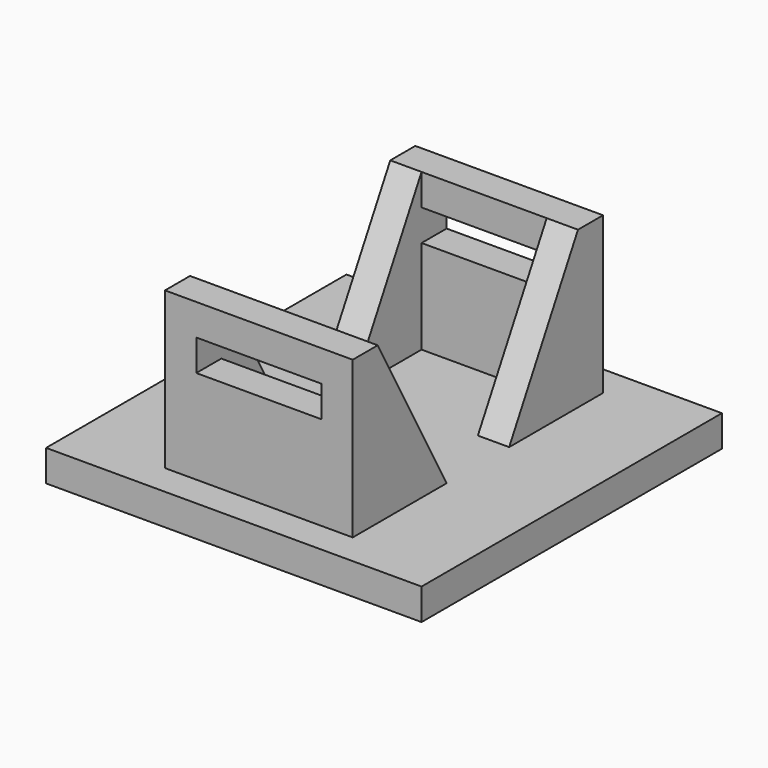
from build123d import *

# Parameters (mm, degrees)
F0_W     = 24
F0_H     = 24
F1_DEPTH = 2
F2_DEPTH = 10
F3_SIZE2 = 9.99999
F3_SIZE  = 5.49999
F4_SIZE2 = 9.99999
F4_SIZE  = 5.49999
F5_W     = 8
F5_H     = 2
F6_DEPTH = 25


# Not quite as in the source:
# - a fillet or chamfer is up to 0.001 mm smaller than in the source, because OpenCascade refuses the exact size


with BuildPart() as f1:
    # F0 (on Top) → F1 (new body)
    with BuildSketch(Plane.XY):
        Rectangle(F0_W, F0_H)
        Polygon((-6, -10), (-6, -2.5), (-4, -2.5), (-4, -8), (0, -8), (4, -8), (4, -2.5), (6, -2.5), (6, -10), (0, -10), align=None, mode=Mode.SUBTRACT)
        Polygon((-4, 2.5), (-6, 2.5), (-6, 10), (0, 10), (6, 10), (6, 2.5), (4, 2.5), (4, 8), (0, 8), (-4, 8), align=None, mode=Mode.SUBTRACT)
        Polygon((-6, 10), (-6, 2.5), (-4, 2.5), (-4, 8), (0, 8), (4, 8), (4, 2.5), (6, 2.5), (6, 10), (0, 10), align=None)
        Polygon((-4, -2.5), (-6, -2.5), (-6, -10), (0, -10), (6, -10), (6, -2.5), (4, -2.5), (4, -8), (0, -8), (-4, -8), align=None)
    extrude(amount=-F1_DEPTH)

    # F0 (on Top) → F2 (join)
    with BuildSketch(Plane.XY):
        Polygon((-6, 10), (-6, 2.5), (-4, 2.5), (-4, 8), (0, 8), (4, 8), (4, 2.5), (6, 2.5), (6, 10), (0, 10), align=None)
        Polygon((-4, -2.5), (-6, -2.5), (-6, -10), (0, -10), (6, -10), (6, -2.5), (4, -2.5), (4, -8), (0, -8), (-4, -8), align=None)
    extrude(amount=F2_DEPTH)

    # F3 (size 5.5 and 10 in the source; OpenCascade refuses exactly that, so slightly less here)
    f3_edges = [f1.edges().sort_by_distance(p)[0] for p in [
        (-5, 2.5, 10),
        (5, 2.5, 10),
    ]]
    f3_side = f1.faces().sort_by_distance((-5.85849, 6.25, 10))[0]
    chamfer(f3_edges, length=F3_SIZE, length2=F3_SIZE2, reference=f3_side)

    # F4 (size 5.5 and 10 in the source; OpenCascade refuses exactly that, so slightly less here)
    f4_edges = [f1.edges().sort_by_distance(p)[0] for p in [
        (5, -2.5, 10),
        (-5, -2.5, 10),
    ]]
    f4_side = f1.faces().sort_by_distance((-5, -2.64151, 10))[0]
    chamfer(f4_edges, length=F4_SIZE, length2=F4_SIZE2, reference=f4_side)

    # F5 (on face) → F6 (cut)
    with BuildSketch(Plane.XZ.offset(10)):
        with Locations((0, 7)):
            Rectangle(F5_W, F5_H)
    extrude(amount=-F6_DEPTH, mode=Mode.SUBTRACT)


solid = f1.part
